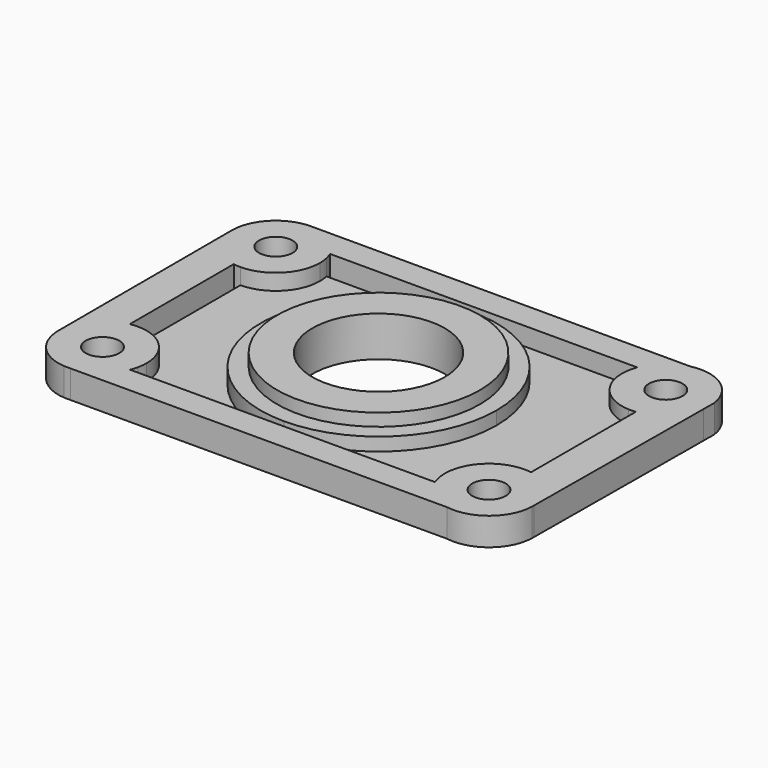
from build123d import *

# Parameters (mm, degrees)
F0_R     = 14.605
F0_R_2   = 9.525
F2_DEPTH = 5.8
F3_DEPTH = 4
F0_R_3   = 2.417765634
F4_DEPTH = 4
F5_DEPTH = 1.7
F6_DEPTH = 0.4


# Not quite as in the source:
# - a feature of the source that left no trace in its solid (it failed there, or was rolled back) is left out


with BuildPart() as f2:
    # F0 (on Top) → F2 (new body)
    with BuildSketch(Plane.XY):
        with Locations((42.1002805233, -21.0943892598)):
            Circle(F0_R)
        with Locations((42.1002805233, -21.0943892598)):
            Circle(F0_R_2, mode=Mode.SUBTRACT)
    extrude(amount=F2_DEPTH)


with BuildPart() as f3:
    # F0 (on Top) → F3 (new body)
    with BuildSketch(Plane.XY):
        with BuildLine():
            ThreePointArc((59.0852805233, -21.0943892598), (54.1104892018, -9.0841805814), (42.1002805233, -4.1093892598))
            ThreePointArc((42.1002805233, -4.1093892598), (25.1152805233, -21.0943892491), (42.1002805018, -38.0793892598))
            ThreePointArc((42.1002805018, -38.0793892598), (54.1104891942, -33.1045979459), (59.0852805233, -21.0943892598))
        make_face()
        with Locations((42.1002805233, -21.0943892598)):
            Circle(F0_R, mode=Mode.SUBTRACT)
    extrude(amount=F3_DEPTH)


with BuildPart() as f4:
    # F0 (on Top) → F4 (new body)
    with BuildSketch(Plane.XY):
        with BuildLine():
            ThreePointArc((70.4796204309, -30.3428000003), (65.5234454038, -32.7230608274), (64.2828575481, -38.0793892598))
            ThreePointArc((64.2828575481, -38.0793892598), (64.4109470876, -38.56194522), (64.5765521859, -39.0329464262))
            ThreePointArc((64.5765521859, -39.0329464262), (66.5006688013, -41.6415820656), (69.4616174351, -42.960668051))
            ThreePointArc((69.4616174351, -42.960668051), (74.513790796, -41.596672905), (76.8261661024, -36.9022231109))
            Line((76.8261661024, -36.9022231109), (76.8285228203, -36.5747387894))
            ThreePointArc((76.8285228203, -36.5747387894), (75.2829744428, -32.5394531286), (71.5131238103, -30.4274691419))
            ThreePointArc((71.5131238103, -30.4274691419), (70.9981033377, -30.3640026837), (70.4796204309, -30.3428000003))
        make_face()
        with Locations((70.4796204309, -36.6928000003)):
            Circle(F0_R_3, mode=Mode.SUBTRACT)
        with BuildLine():
            ThreePointArc((77.0462929913, -6.3138761602), (75.1657734813, -9.8791990856), (71.5131238103, -11.5839077326))
            Line((71.5131238103, -11.5839077326), (71.5131238103, -30.4274691419))
            ThreePointArc((71.5131238103, -30.4274691419), (75.2829744428, -32.5394531286), (76.8285228203, -36.5747387894))
            Line((76.8285228203, -36.5747387894), (77.0462929913, -6.3138761602))
        make_face()
        with BuildLine():
            ThreePointArc((69.4468072263, 0.8754916674), (66.6800084328, -0.5074468562), (64.9001725386, -3.0372450128))
            ThreePointArc((64.9001725386, -3.0372450128), (64.7236558931, -3.5665671194), (64.5944887824, -4.1093892598))
            ThreePointArc((64.5944887824, -4.1093892598), (65.8285113374, -9.2019743288), (70.4796204309, -11.6153575458))
            ThreePointArc((70.4796204309, -11.6153575458), (70.9970160236, -11.6207925725), (71.5131238103, -11.5839077326))
            ThreePointArc((71.5131238103, -11.5839077326), (75.1657734813, -9.8791990856), (77.0462929913, -6.3138761602))
            Line((77.0462929913, -6.3138761602), (77.0602332407, -4.3767698617))
            ThreePointArc((77.0602332407, -4.3767698617), (74.3954165151, -0.0954010996), (69.4468072263, 0.8754916674))
        make_face()
        with Locations((70.8046832573, -5.3003555452)):
            Circle(F0_R_3, mode=Mode.SUBTRACT)
        with BuildLine():
            ThreePointArc((14.8128727451, 0.8754916674), (18.3374917259, -0.1925048263), (20.6765104821, -3.0372450128))
            Line((20.6765104821, -3.0372450128), (64.9001725386, -3.0372450128))
            ThreePointArc((64.9001725386, -3.0372450128), (66.6800084328, -0.5074468562), (69.4468072263, 0.8754916674))
            Line((69.4468072263, 0.8754916674), (14.8128727451, 0.8754916674))
        make_face()
        with BuildLine():
            ThreePointArc((14.8128727451, -11.8245083326), (19.3030008056, -9.9646363931), (21.1628727451, -5.4745083326))
            ThreePointArc((21.1628727451, -5.4745083326), (21.1256456301, -4.7879236676), (21.0144007759, -4.1093892598))
            ThreePointArc((21.0144007759, -4.1093892598), (20.8692272239, -3.5658254287), (20.6765104821, -3.0372450128))
            ThreePointArc((20.6765104821, -3.0372450128), (18.3374917259, -0.1925048263), (14.8128727451, 0.8754916674))
            ThreePointArc((14.8128727451, 0.8754916674), (10.3227446846, -0.984380272), (8.4628727451, -5.4745083326))
            ThreePointArc((8.4628727451, -5.4745083326), (9.9708557742, -9.5827161722), (13.7785803527, -11.7397089875))
            ThreePointArc((13.7785803527, -11.7397089875), (14.2939913324, -11.8032729892), (14.8128727451, -11.8245083326))
        make_face()
        with Locations((14.8128727451, -5.4745083326)):
            Circle(F0_R_3, mode=Mode.SUBTRACT)
        with BuildLine():
            ThreePointArc((13.7785803527, -11.7397089875), (9.9708557742, -9.5827161722), (8.4628727451, -5.4745083326))
            Line((8.4628727451, -5.4745083326), (8.5004888147, -36.7004494693))
            ThreePointArc((8.5004888147, -36.7004494693), (9.9936868257, -32.6020764465), (13.7785803527, -30.4339245321))
            Line((13.7785803527, -30.4339245321), (13.7785803527, -11.7397089875))
        make_face()
        with BuildLine():
            ThreePointArc((21.2004842073, -36.6928000003), (19.3272948586, -32.1893939124), (14.8128727451, -30.3429113889))
            ThreePointArc((14.8128727451, -30.3429113889), (14.2938632343, -30.3672428634), (13.7785803527, -30.4339245321))
            ThreePointArc((13.7785803527, -30.4339245321), (9.9936868257, -32.6020764465), (8.5004888147, -36.7004494693))
            ThreePointArc((8.5004888147, -36.7004494693), (10.207762887, -41.024963287), (14.4039206737, -43.0270782552))
            Line((14.4039206737, -43.0270782552), (15.3123271424, -43.0259825418))
            ThreePointArc((15.3123271424, -43.0259825418), (18.5830125205, -41.8299910996), (20.7310672048, -39.0888892326))
            ThreePointArc((20.7310672048, -39.0888892326), (20.9102155072, -38.5907348182), (21.0472470901, -38.0793892598))
            ThreePointArc((21.0472470901, -38.0793892598), (21.1620586664, -37.390315482), (21.2004842073, -36.6928000003))
        make_face()
        with Locations((14.8504842073, -36.6928000003)):
            Circle(F0_R_3, mode=Mode.SUBTRACT)
        with BuildLine():
            Line((64.5765521859, -39.0329464262), (20.7310672048, -39.0888892326))
            ThreePointArc((20.7310672048, -39.0888892326), (18.5830125205, -41.8299910996), (15.3123271424, -43.0259825418))
            Line((15.3123271424, -43.0259825418), (69.4616174351, -42.960668051))
            ThreePointArc((69.4616174351, -42.960668051), (66.5006688013, -41.6415820656), (64.5765521859, -39.0329464262))
        make_face()
    extrude(amount=F4_DEPTH)


with BuildPart() as f5:
    # F0 (on Top) → F5 (new body)
    with BuildSketch(Plane.XY):
        with BuildLine():
            ThreePointArc((21.0144007759, -4.1093892598), (21.1256456301, -4.7879236676), (21.1628727451, -5.4745083326))
            ThreePointArc((21.1628727451, -5.4745083326), (19.3030008056, -9.9646363931), (14.8128727451, -11.8245083326))
            Line((14.8128727451, -11.8245083326), (14.8128727451, -30.3429113889))
            ThreePointArc((14.8128727451, -30.3429113889), (19.3272948586, -32.1893939124), (21.2004842073, -36.6928000003))
            ThreePointArc((21.2004842073, -36.6928000003), (21.1620586664, -37.390315482), (21.0472470901, -38.0793892598))
            Line((21.0472470901, -38.0793892598), (42.1002805018, -38.0793892598))
            ThreePointArc((42.1002805018, -38.0793892598), (25.1152805233, -21.0943892491), (42.1002805233, -4.1093892598))
            Line((42.1002805233, -4.1093892598), (21.0144007759, -4.1093892598))
        make_face()
    extrude(amount=F5_DEPTH)


with BuildPart() as f5b:
    # F0 (on Top) → F5, piece 2 (new body)
    with BuildSketch(Plane.XY):
        with BuildLine():
            Line((64.5944887824, -4.1093892598), (42.1002805233, -4.1093892598))
            ThreePointArc((42.1002805233, -4.1093892598), (54.1104892018, -9.0841805814), (59.0852805233, -21.0943892598))
            ThreePointArc((59.0852805233, -21.0943892598), (54.1104891942, -33.1045979459), (42.1002805018, -38.0793892598))
            Line((42.1002805018, -38.0793892598), (64.2828575481, -38.0793892598))
            ThreePointArc((64.2828575481, -38.0793892598), (65.5234454038, -32.7230608274), (70.4796204309, -30.3428000003))
            Line((70.4796204309, -30.3428000003), (70.4796204309, -11.6153575458))
            ThreePointArc((70.4796204309, -11.6153575458), (65.8285113374, -9.2019743288), (64.5944887824, -4.1093892598))
        make_face()
    extrude(amount=F5_DEPTH)


with BuildPart() as f6:
    # F6 (new): a face of the model
    f6_faces = [f5b.part.faces().sort_by_distance(p)[0] for p in [
        (61.5462800448, -20.981916528, 1.7),
    ]]
    extrude(f6_faces, amount=F6_DEPTH)


solid = Compound([f2.part, f3.part, f4.part, f5.part, f5b.part, f6.part])
